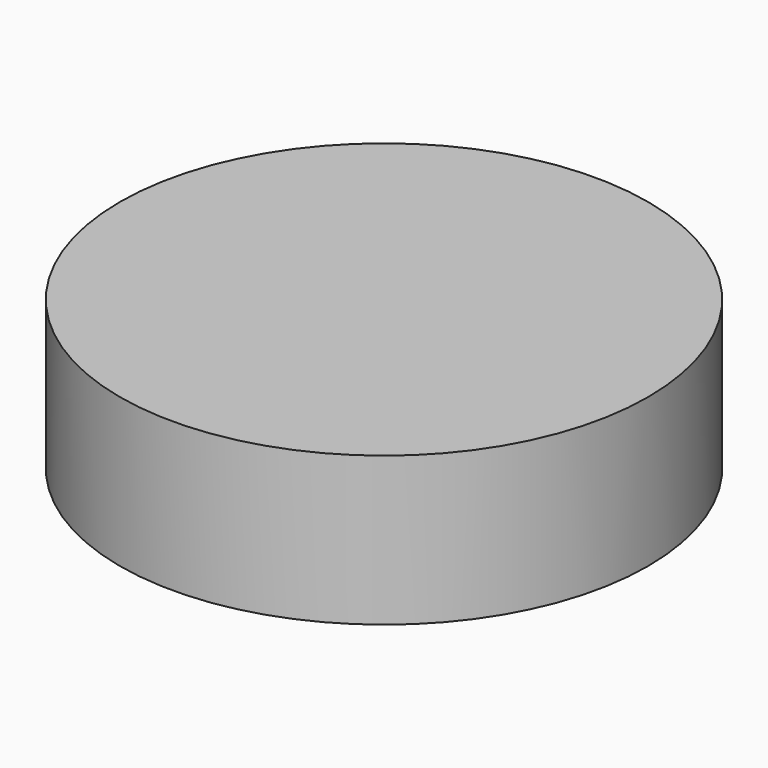
from build123d import *

# Parameters (mm, degrees)
F0_R     = 22.5416252379
F2_DEPTH = 12.7
F3_R     = 22.6896174347
F4_DEPTH = 2.54


# Not quite as in the source:
# - the program builds the solid bodies; features that only make, move or delete a surface that nothing else refers to are left out


with BuildPart() as f2:
    # F0 (on Top) → F2 (new body)
    with BuildSketch(Plane.XY):
        Circle(F0_R)
    extrude(amount=F2_DEPTH)

    # F3 (on Top) → F4 (cut)
    with BuildSketch(Plane.XY):
        Circle(F3_R)
    extrude(amount=-F4_DEPTH, mode=Mode.SUBTRACT)


solid = f2.part
